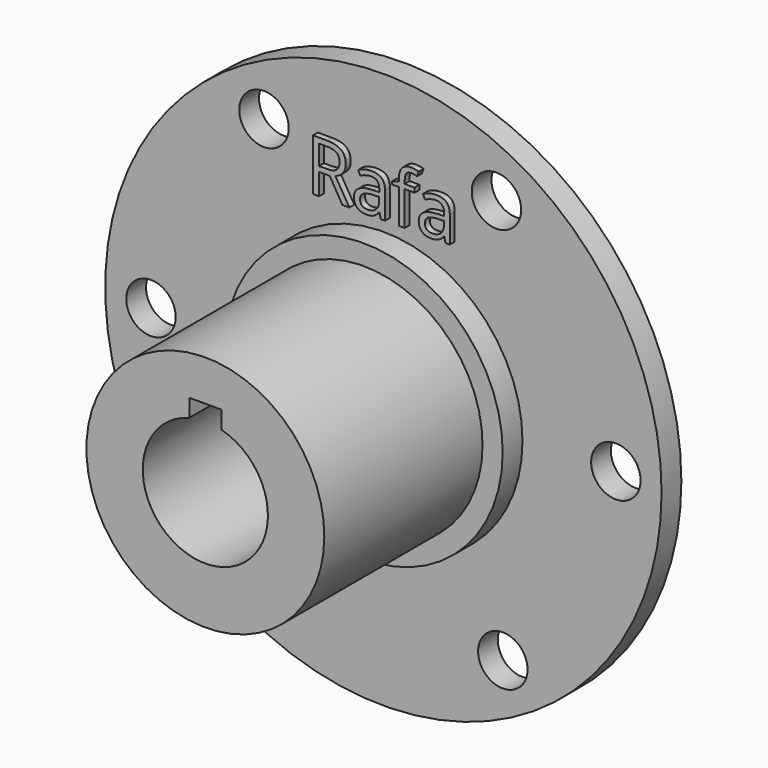
from build123d import *

# Parameters (mm, degrees)
F0_R         = 28.575
F0_R_2       = 2.54
F0_R_3       = 14.2875
F1_DEPTH     = 2.54
F0_R_4       = 12.2174
F2_DEPTH     = 5.08
F3_DEPTH     = 25.4
F4_TEXT_SIZE = 7.4338245516
F5_DEPTH     = 3.175


# Not quite as in the source:
# - Text() gives the source's letters only with a copy of the font that has no kerning and outlines rounded to 1/6400 em; it was checked with that copy


with BuildPart() as f1:
    # F0 (on Front) → F1 (new body)
    with BuildSketch(Plane.XZ):
        Circle(F0_R)
        with Locations((-11.611554856, -20.8671413431)):
            Circle(F0_R_2, mode=Mode.SUBTRACT)
        with Locations((-23.8772519354, -0.3776691888)):
            Circle(F0_R_2, mode=Mode.SUBTRACT)
        with Locations((12.2656970795, -20.4894721542)):
            Circle(F0_R_2, mode=Mode.SUBTRACT)
        with Locations((-12.2656970795, 20.4894721542)):
            Circle(F0_R_2, mode=Mode.SUBTRACT)
        Circle(F0_R_3, mode=Mode.SUBTRACT)
        with Locations((23.8772519355, 0.3776691888)):
            Circle(F0_R_2, mode=Mode.SUBTRACT)
        with Locations((11.611554856, 20.8671413431)):
            Circle(F0_R_2, mode=Mode.SUBTRACT)
    extrude(amount=F1_DEPTH)

    # F0 (on Front) → F2 (join)
    with BuildSketch(Plane.XZ):
        Circle(F0_R_3)
        Circle(F0_R_4, mode=Mode.SUBTRACT)
    extrude(amount=F2_DEPTH)

    # F0 (on Front) → F3 (join)
    with BuildSketch(Plane.XZ):
        Circle(F0_R_4)
        with BuildLine():
            ThreePointArc((1.651, 6.2104947822), (0, -6.4262), (-1.651, 6.2104947822))
            Line((-1.651, 6.2104947822), (-1.651, 8.0264))
            Line((-1.651, 8.0264), (1.651, 8.0264))
            Line((1.651, 8.0264), (1.651, 6.2104947822))
        make_face(mode=Mode.SUBTRACT)
    extrude(amount=F3_DEPTH)

    # F4 (on Front) → F5 (join)
    with BuildSketch(Plane.XZ):
        with Locations((-7.4519538321, 15.759431757)):
            Text('Rafa', F4_TEXT_SIZE, font='Open Sans', text_align=(TextAlign.LEFT, TextAlign.BOTTOM))
    extrude(amount=F5_DEPTH)


solid = f1.part
